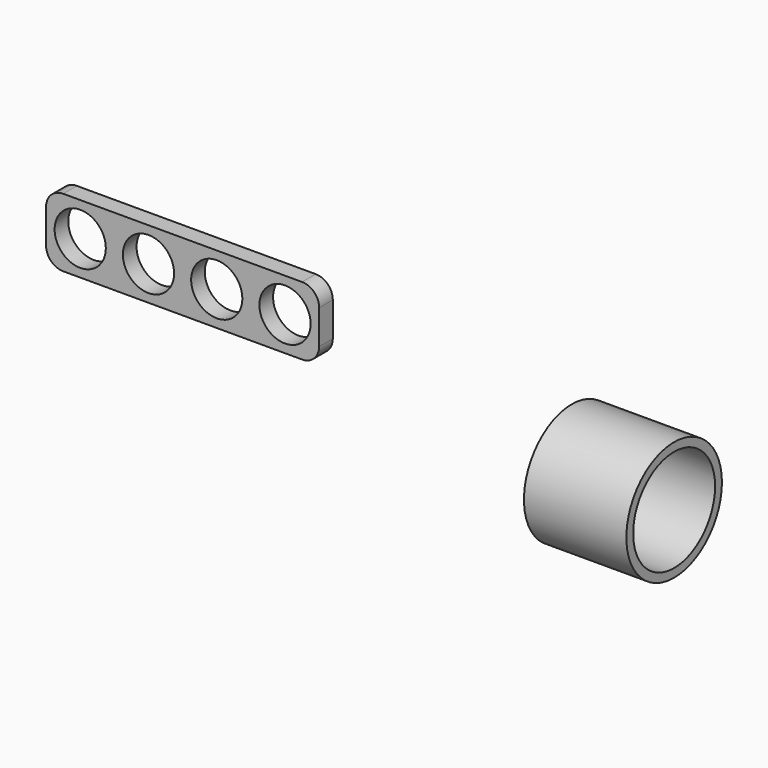
from build123d import *

# Parameters (mm, degrees)
F0_R     = 37.5
F1_DEPTH = 25
F3_R     = 87.5
F3_R_2   = 75
F4_DEPTH = 150


# Not quite as in the source:
# - the program builds the solid bodies; features that only make, move or delete a surface that nothing else refers to are left out


with BuildPart() as f1:
    # F0 (on Front) → F1 (new body)
    with BuildSketch(Plane.XZ):
        with BuildLine():
            ThreePointArc((250, 25), (242.6776695297, 42.6776695297), (225, 50))
            Line((225, 50), (-125, 50))
            ThreePointArc((-125, 50), (-142.6776695297, 42.6776695297), (-150, 25))
            Line((-150, 25), (-150, -25))
            ThreePointArc((-150, -25), (-142.6776695297, -42.6776695297), (-125, -50))
            Line((-125, -50), (225, -50))
            ThreePointArc((225, -50), (242.6776695297, -42.6776695297), (250, -25))
            Line((250, -25), (250, 25))
        make_face()
        with Locations((-100, 0)):
            Circle(F0_R, mode=Mode.SUBTRACT)
        Circle(F0_R, mode=Mode.SUBTRACT)
        with Locations((100, 0)):
            Circle(F0_R, mode=Mode.SUBTRACT)
        with Locations((200, 0)):
            Circle(F0_R, mode=Mode.SUBTRACT)
    extrude(amount=F1_DEPTH)


with BuildPart() as f4:
    # F3 (on offset) → F4 (new body)
    with BuildSketch(Plane.YZ.offset(400)):
        with Locations((250, -250)):
            Circle(F3_R)
        with Locations((250, -250)):
            Circle(F3_R_2, mode=Mode.SUBTRACT)
    extrude(amount=F4_DEPTH)


solid = Compound([f1.part, f4.part])
